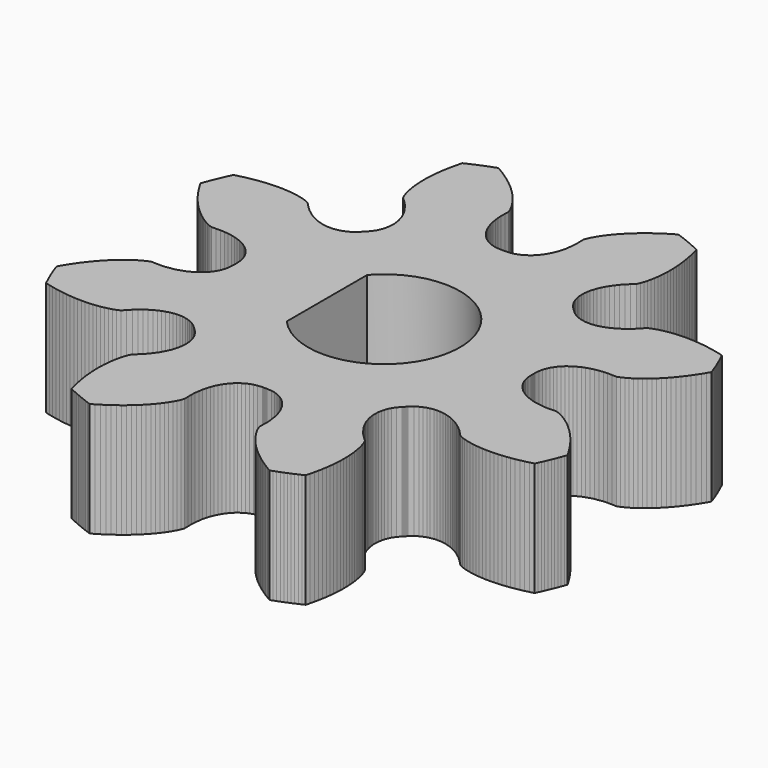
from build123d import *

# Parameters (mm, degrees)
F1_DEPTH = 3


# Not quite as in the source:
# - ends of sketch curves that miss each other by under 0.0002 mm in the source are joined


with BuildPart() as f1:
    # F0 (on Top) → F1 (new body)
    with BuildSketch(Plane.XY):
        Polygon((3.91873, -0.01261), (3.91875, 0), (3.91873, 0.01261), (3.918669, 0.02522), (3.918567, 0.037829), (3.918425, 0.050438), (3.918243, 0.063047), (3.927022, 0.180894), (3.946465, 0.280905), (3.974611, 0.359921), (4.009085, 0.438851), (4.050739, 0.504778), (4.097447, 0.573512), (4.150796, 0.631412), (4.209027, 0.689888), (4.273539, 0.739418), (4.342741, 0.789047), (4.418306, 0.828977), (4.498112, 0.870334), (4.584187, 0.902056), (4.674962, 0.93187), (4.771145, 0.955731), (4.873257, 0.970539), (4.979177, 0.986368), (5.091067, 0.991698), (5.208217, 0.989239), (5.32907, 0.986364), (5.410163, 1.016651), (5.489651, 1.055105), (5.56805, 1.098614), (5.64541, 1.146577), (5.721741, 1.198614), (5.797032, 1.254457), (5.87126, 1.313903), (5.944393, 1.376794), (6.016393, 1.443001), (6.08722, 1.512416), (6.15683, 1.584946), (6.225176, 1.660508), (6.292211, 1.739031), (6.357886, 1.820446), (6.42215, 1.904693), (6.484952, 1.991715), (6.546241, 2.081459), (6.605965, 2.173872), (6.664072, 2.268905), (6.72051, 2.36651), (6.694499, 2.43912), (6.667703, 2.511445), (6.640127, 2.583475), (6.611771, 2.655203), (6.582642, 2.726619), (6.5527401565, 2.797716063), (6.5220715212, 2.8684861381), (6.4906377963, 2.9389182162), (6.4584439317, 3.0090073474), (6.4254934628, 3.0787429253), (6.3165686129, 3.1078523901), (6.2082822804, 3.1339630151), (6.100705176, 3.1570776287), (5.9939087176, 3.1771983522), (5.8879671512, 3.1943244784), (5.782954016, 3.2084545932), (5.6789456796, 3.219584454), (5.5760206307, 3.2277076967), (5.474262308, 3.2328101792), (5.3737541501, 3.234874931), (5.2745880809, 3.2338764962), (5.176860974, 3.2297802266), (5.0806774812, 3.222538039), (4.9861556894, 3.2120855865), (4.8934299487, 3.1983337739), (4.8026600654, 3.1811553217), (4.7140433223, 3.1603685037), (4.6278413488, 3.1356975481), (4.5444437608, 3.1066821284), (4.4656862075, 3.0707568613), (4.3822631637, 2.9832679535), (4.3011643799, 2.8986916185), (4.218277323, 2.8233423199), (4.1321877795, 2.7596383629), (4.0495128546, 2.6979051124), (3.9646289282, 2.6467657358), (3.8793596285, 2.6036597993), (3.796064571, 2.5652264244), (3.7103893921, 2.5380388758), (3.6287220944, 2.5128411257), (3.5446958885, 2.4990009246), (3.464056017, 2.4884070508), (3.3815317058, 2.488580292), (3.3028667835, 2.491798335), (3.2212369625, 2.5073730689), (3.1451657079, 2.5245366718), (3.0649769705, 2.5559718109), (2.9892019936, 2.5919423328), (2.9047352601, 2.648912512), (2.8151971569, 2.7260352344), (2.8064099409, 2.7350798372), (2.7975944407, 2.7440961558), (2.7887506561, 2.7530841901), (2.7798771732, 2.7620439401), (2.7709746988, 2.7709746988), (2.7620439401, 2.7798771732), (2.7530841901, 2.7887506561), (2.7440961558, 2.7975944407), (2.7350798372, 2.8064099409), (2.7260352344, 2.8151971569), (2.648912512, 2.9047352601), (2.5919423328, 2.9892019936), (2.5559718109, 3.0649769705), (2.5245366718, 3.1451657079), (2.5073730689, 3.2212369625), (2.491798335, 3.3028667835), (2.488580292, 3.3815317058), (2.4884070508, 3.464056017), (2.4990009246, 3.5446958885), (2.5128411257, 3.6287220944), (2.5380388758, 3.7103893921), (2.5652264244, 3.796064571), (2.6036597993, 3.8793596285), (2.6467657358, 3.9646289282), (2.6979051124, 4.0495128546), (2.7596383629, 4.1321877795), (2.8233423199, 4.218277323), (2.8986916185, 4.3011643799), (2.9832679535, 4.3822631637), (3.0707568613, 4.4656862075), (3.1066821284, 4.5444437608), (3.1356975481, 4.6278413488), (3.1603685037, 4.7140433223), (3.1811553217, 4.8026600654), (3.1983337739, 4.8934299487), (3.2120855865, 4.9861556894), (3.222538039, 5.0806774812), (3.2297802266, 5.176860974), (3.2338764962, 5.2745880809), (3.234874931, 5.3737541501), (3.2328101792, 5.474262308), (3.2277076967, 5.5760206307), (3.219584454, 5.6789456796), (3.2084545932, 5.782954016), (3.1943244784, 5.8879671512), (3.1771983522, 5.9939087176), (3.1570776287, 6.100705176), (3.1339630151, 6.2082822804), (3.1078523901, 6.3165686129), (3.0787429253, 6.4254934628), (3.0090073474, 6.4584439317), (2.9389182162, 6.4906377963), (2.8684861381, 6.5220715212), (2.797716063, 6.5527401565), (2.7266200117, 6.5826415809), (2.655203, 6.611771), (2.583475, 6.640127), (2.511445, 6.667703), (2.43912, 6.694499), (2.36651, 6.72051), (2.268905, 6.664072), (2.173872, 6.605965), (2.081459, 6.546241), (1.991715, 6.484952), (1.904693, 6.42215), (1.820446, 6.357886), (1.739031, 6.292211), (1.660508, 6.225176), (1.584946, 6.15683), (1.512416, 6.08722), (1.443001, 6.016393), (1.376794, 5.944393), (1.313903, 5.87126), (1.254457, 5.797032), (1.198614, 5.721741), (1.146577, 5.64541), (1.098614, 5.56805), (1.055105, 5.489651), (1.016651, 5.410163), (0.986364, 5.32907), (0.989239, 5.208217), (0.991698, 5.091067), (0.986368, 4.979177), (0.970539, 4.873257), (0.955731, 4.771145), (0.93187, 4.674962), (0.902056, 4.584187), (0.870334, 4.498112), (0.828977, 4.418306), (0.789047, 4.342741), (0.739418, 4.273539), (0.689888, 4.209027), (0.631412, 4.150796), (0.573512, 4.097447), (0.504778, 4.050739), (0.438851, 4.009085), (0.359921, 3.974611), (0.280905, 3.946465), (0.180894, 3.927022), (0.063047, 3.918243), (0.050438, 3.918425), (0.037829, 3.918567), (0.02522, 3.918669), (0.01261, 3.91873), (0, 3.91875), (-0.01261, 3.91873), (-0.02522, 3.918669), (-0.037829, 3.918567), (-0.050438, 3.918425), (-0.063047, 3.918243), (-0.180894, 3.927022), (-0.280905, 3.946465), (-0.359921, 3.974611), (-0.438851, 4.009085), (-0.504778, 4.050739), (-0.573512, 4.097447), (-0.631412, 4.150796), (-0.689888, 4.209027), (-0.739418, 4.273539), (-0.789047, 4.342741), (-0.828977, 4.418306), (-0.870334, 4.498112), (-0.902056, 4.584187), (-0.93187, 4.674962), (-0.955731, 4.771145), (-0.970539, 4.873257), (-0.986368, 4.979177), (-0.991698, 5.091067), (-0.989239, 5.208217), (-0.986364, 5.32907), (-1.016651, 5.410163), (-1.055105, 5.489651), (-1.098614, 5.56805), (-1.146577, 5.64541), (-1.198614, 5.721741), (-1.254457, 5.797032), (-1.313903, 5.87126), (-1.376794, 5.944393), (-1.443001, 6.016393), (-1.512416, 6.08722), (-1.584946, 6.15683), (-1.660508, 6.225176), (-1.739031, 6.292211), (-1.820446, 6.357886), (-1.904693, 6.42215), (-1.991715, 6.484952), (-2.081459, 6.546241), (-2.173872, 6.605965), (-2.268905, 6.664072), (-2.36651, 6.72051), (-2.43912, 6.694499), (-2.511445, 6.667703), (-2.583475, 6.640127), (-2.655203, 6.611771), (-2.726619, 6.582642), (-2.797716063, 6.5527401565), (-2.8684861381, 6.5220715212), (-2.9389182162, 6.4906377963), (-3.0090073474, 6.4584439317), (-3.0787429253, 6.4254934628), (-3.1078523901, 6.3165686129), (-3.1339630151, 6.2082822804), (-3.1570776287, 6.100705176), (-3.1771983522, 5.9939087176), (-3.1943244784, 5.8879671512), (-3.2084545932, 5.782954016), (-3.219584454, 5.6789456796), (-3.2277076967, 5.5760206307), (-3.2328101792, 5.474262308), (-3.234874931, 5.3737541501), (-3.2338764962, 5.2745880809), (-3.2297802266, 5.176860974), (-3.222538039, 5.0806774812), (-3.2120855865, 4.9861556894), (-3.1983337739, 4.8934299487), (-3.1811553217, 4.8026600654), (-3.1603685037, 4.7140433223), (-3.1356975481, 4.6278413488), (-3.1066821284, 4.5444437608), (-3.0707568613, 4.4656862075), (-2.9832679535, 4.3822631637), (-2.8986916185, 4.3011643799), (-2.8233423199, 4.218277323), (-2.7596383629, 4.1321877795), (-2.6979051124, 4.0495128546), (-2.6467657358, 3.9646289282), (-2.6036597993, 3.8793596285), (-2.5652264244, 3.796064571), (-2.5380388758, 3.7103893921), (-2.5128411257, 3.6287220944), (-2.4990009246, 3.5446958885), (-2.4884070508, 3.464056017), (-2.488580292, 3.3815317058), (-2.491798335, 3.3028667835), (-2.5073730689, 3.2212369625), (-2.5245366718, 3.1451657079), (-2.5559718109, 3.0649769705), (-2.5919423328, 2.9892019936), (-2.648912512, 2.9047352601), (-2.7260352344, 2.8151971569), (-2.7350798372, 2.8064099409), (-2.7440961558, 2.7975944407), (-2.7530841901, 2.7887506561), (-2.7620439401, 2.7798771732), (-2.7709746988, 2.7709746988), (-2.7798771732, 2.7620439401), (-2.7887506561, 2.7530841901), (-2.7975944407, 2.7440961558), (-2.8064099409, 2.7350798372), (-2.8151971569, 2.7260352344), (-2.9047352601, 2.648912512), (-2.9892019936, 2.5919423328), (-3.0649769705, 2.5559718109), (-3.1451657079, 2.5245366718), (-3.2212369625, 2.5073730689), (-3.3028667835, 2.491798335), (-3.3815317058, 2.488580292), (-3.464056017, 2.4884070508), (-3.5446958885, 2.4990009246), (-3.6287220944, 2.5128411257), (-3.7103893921, 2.5380388758), (-3.796064571, 2.5652264244), (-3.8793596285, 2.6036597993), (-3.9646289282, 2.6467657358), (-4.0495128546, 2.6979051124), (-4.1321877795, 2.7596383629), (-4.218277323, 2.8233423199), (-4.3011643799, 2.8986916185), (-4.3822631637, 2.9832679535), (-4.4656862075, 3.0707568613), (-4.5444437608, 3.1066821284), (-4.6278413488, 3.1356975481), (-4.7140433223, 3.1603685037), (-4.8026600654, 3.1811553217), (-4.8934299487, 3.1983337739), (-4.9861556894, 3.2120855865), (-5.0806774812, 3.222538039), (-5.176860974, 3.2297802266), (-5.2745880809, 3.2338764962), (-5.3737541501, 3.234874931), (-5.474262308, 3.2328101792), (-5.5760206307, 3.2277076967), (-5.6789456796, 3.219584454), (-5.782954016, 3.2084545932), (-5.8879671512, 3.1943244784), (-5.9939087176, 3.1771983522), (-6.100705176, 3.1570776287), (-6.2082822804, 3.1339630151), (-6.3165686129, 3.1078523901), (-6.4254934628, 3.0787429253), (-6.4584439317, 3.0090073474), (-6.4906377963, 2.9389182162), (-6.5220715212, 2.8684861381), (-6.5527401565, 2.797716063), (-6.5826415809, 2.7266200117), (-6.611771, 2.655203), (-6.640127, 2.583475), (-6.667703, 2.511445), (-6.694499, 2.43912), (-6.72051, 2.36651), (-6.664072, 2.268905), (-6.605965, 2.173872), (-6.546241, 2.081459), (-6.484952, 1.991715), (-6.42215, 1.904693), (-6.357886, 1.820446), (-6.292211, 1.739031), (-6.225176, 1.660508), (-6.15683, 1.584946), (-6.08722, 1.512416), (-6.016393, 1.443001), (-5.944393, 1.376794), (-5.87126, 1.313903), (-5.797032, 1.254457), (-5.721741, 1.198614), (-5.64541, 1.146577), (-5.56805, 1.098614), (-5.489651, 1.055105), (-5.410163, 1.016651), (-5.32907, 0.986364), (-5.208217, 0.989239), (-5.091067, 0.991698), (-4.979177, 0.986368), (-4.873257, 0.970539), (-4.771145, 0.955731), (-4.674962, 0.93187), (-4.584187, 0.902056), (-4.498112, 0.870334), (-4.418306, 0.828977), (-4.342741, 0.789047), (-4.273539, 0.739418), (-4.209027, 0.689888), (-4.150796, 0.631412), (-4.097447, 0.573512), (-4.050739, 0.504778), (-4.009085, 0.438851), (-3.974611, 0.359921), (-3.946465, 0.280905), (-3.927022, 0.180894), (-3.918243, 0.063047), (-3.918425, 0.050438), (-3.918567, 0.037829), (-3.918669, 0.02522), (-3.91873, 0.01261), (-3.91875, 0), (-3.91873, -0.01261), (-3.918669, -0.02522), (-3.918567, -0.037829), (-3.918425, -0.050438), (-3.918243, -0.063047), (-3.927022, -0.180894), (-3.946465, -0.280905), (-3.974611, -0.359921), (-4.009085, -0.438851), (-4.050739, -0.504778), (-4.097447, -0.573512), (-4.150796, -0.631412), (-4.209027, -0.689888), (-4.273539, -0.739418), (-4.342741, -0.789047), (-4.418306, -0.828977), (-4.498112, -0.870334), (-4.584187, -0.902056), (-4.674962, -0.93187), (-4.771145, -0.955731), (-4.873257, -0.970539), (-4.979177, -0.986368), (-5.091067, -0.991698), (-5.208217, -0.989239), (-5.32907, -0.986364), (-5.410163, -1.016651), (-5.489651, -1.055105), (-5.56805, -1.098614), (-5.64541, -1.146577), (-5.721741, -1.198614), (-5.797032, -1.254457), (-5.87126, -1.313903), (-5.944393, -1.376794), (-6.016393, -1.443001), (-6.08722, -1.512416), (-6.15683, -1.584946), (-6.225176, -1.660508), (-6.292211, -1.739031), (-6.357886, -1.820446), (-6.42215, -1.904693), (-6.484952, -1.991715), (-6.546241, -2.081459), (-6.605965, -2.173872), (-6.664072, -2.268905), (-6.72051, -2.36651), (-6.694499, -2.43912), (-6.667703, -2.511445), (-6.640127, -2.583475), (-6.611771, -2.655203), (-6.582642, -2.726619), (-6.5527401565, -2.797716063), (-6.5220715212, -2.8684861381), (-6.4906377963, -2.9389182162), (-6.4584439317, -3.0090073474), (-6.4254934628, -3.0787429253), (-6.3165686129, -3.1078523901), (-6.2082822804, -3.1339630151), (-6.100705176, -3.1570776287), (-5.9939087176, -3.1771983522), (-5.8879671512, -3.1943244784), (-5.782954016, -3.2084545932), (-5.6789456796, -3.219584454), (-5.5760206307, -3.2277076967), (-5.474262308, -3.2328101792), (-5.3737541501, -3.234874931), (-5.2745880809, -3.2338764962), (-5.176860974, -3.2297802266), (-5.0806774812, -3.222538039), (-4.9861556894, -3.2120855865), (-4.8934299487, -3.1983337739), (-4.8026600654, -3.1811553217), (-4.7140433223, -3.1603685037), (-4.6278413488, -3.1356975481), (-4.5444437608, -3.1066821284), (-4.4656862075, -3.0707568613), (-4.3822631637, -2.9832679535), (-4.3011643799, -2.8986916185), (-4.218277323, -2.8233423199), (-4.1321877795, -2.7596383629), (-4.0495128546, -2.6979051124), (-3.9646289282, -2.6467657358), (-3.8793596285, -2.6036597993), (-3.796064571, -2.5652264244), (-3.7103893921, -2.5380388758), (-3.6287220944, -2.5128411257), (-3.5446958885, -2.4990009246), (-3.464056017, -2.4884070508), (-3.3815317058, -2.488580292), (-3.3028667835, -2.491798335), (-3.2212369625, -2.5073730689), (-3.1451657079, -2.5245366718), (-3.0649769705, -2.5559718109), (-2.9892019936, -2.5919423328), (-2.9047352601, -2.648912512), (-2.8151971569, -2.7260352344), (-2.8064099409, -2.7350798372), (-2.7975944407, -2.7440961558), (-2.7887506561, -2.7530841901), (-2.7798771732, -2.7620439401), (-2.7709746988, -2.7709746988), (-2.7620439401, -2.7798771732), (-2.7530841901, -2.7887506561), (-2.7440961558, -2.7975944407), (-2.7350798372, -2.8064099409), (-2.7260352344, -2.8151971569), (-2.648912512, -2.9047352601), (-2.5919423328, -2.9892019936), (-2.5559718109, -3.0649769705), (-2.5245366718, -3.1451657079), (-2.5073730689, -3.2212369625), (-2.491798335, -3.3028667835), (-2.488580292, -3.3815317058), (-2.4884070508, -3.464056017), (-2.4990009246, -3.5446958885), (-2.5128411257, -3.6287220944), (-2.5380388758, -3.7103893921), (-2.5652264244, -3.796064571), (-2.6036597993, -3.8793596285), (-2.6467657358, -3.9646289282), (-2.6979051124, -4.0495128546), (-2.7596383629, -4.1321877795), (-2.8233423199, -4.218277323), (-2.8986916185, -4.3011643799), (-2.9832679535, -4.3822631637), (-3.0707568613, -4.4656862075), (-3.1066821284, -4.5444437608), (-3.1356975481, -4.6278413488), (-3.1603685037, -4.7140433223), (-3.1811553217, -4.8026600654), (-3.1983337739, -4.8934299487), (-3.2120855865, -4.9861556894), (-3.222538039, -5.0806774812), (-3.2297802266, -5.176860974), (-3.2338764962, -5.2745880809), (-3.234874931, -5.3737541501), (-3.2328101792, -5.474262308), (-3.2277076967, -5.5760206307), (-3.219584454, -5.6789456796), (-3.2084545932, -5.782954016), (-3.1943244784, -5.8879671512), (-3.1771983522, -5.9939087176), (-3.1570776287, -6.100705176), (-3.1339630151, -6.2082822804), (-3.1078523901, -6.3165686129), (-3.0787429253, -6.4254934628), (-3.0090073474, -6.4584439317), (-2.9389182162, -6.4906377963), (-2.8684861381, -6.5220715212), (-2.797716063, -6.5527401565), (-2.7266200117, -6.5826415809), (-2.655203, -6.611771), (-2.583475, -6.640127), (-2.511445, -6.667703), (-2.43912, -6.694499), (-2.36651, -6.72051), (-2.268905, -6.664072), (-2.173872, -6.605965), (-2.081459, -6.546241), (-1.991715, -6.484952), (-1.904693, -6.42215), (-1.820446, -6.357886), (-1.739031, -6.292211), (-1.660508, -6.225176), (-1.584946, -6.15683), (-1.512416, -6.08722), (-1.443001, -6.016393), (-1.376794, -5.944393), (-1.313903, -5.87126), (-1.254457, -5.797032), (-1.198614, -5.721741), (-1.146577, -5.64541), (-1.098614, -5.56805), (-1.055105, -5.489651), (-1.016651, -5.410163), (-0.986364, -5.32907), (-0.989239, -5.208217), (-0.991698, -5.091067), (-0.986368, -4.979177), (-0.970539, -4.873257), (-0.955731, -4.771145), (-0.93187, -4.674962), (-0.902056, -4.584187), (-0.870334, -4.498112), (-0.828977, -4.418306), (-0.789047, -4.342741), (-0.739418, -4.273539), (-0.689888, -4.209027), (-0.631412, -4.150796), (-0.573512, -4.097447), (-0.504778, -4.050739), (-0.438851, -4.009085), (-0.359921, -3.974611), (-0.280905, -3.946465), (-0.180894, -3.927022), (-0.063047, -3.918243), (-0.050438, -3.918425), (-0.037829, -3.918567), (-0.02522, -3.918669), (-0.01261, -3.91873), (0, -3.91875), (0.01261, -3.91873), (0.02522, -3.918669), (0.037829, -3.918567), (0.050438, -3.918425), (0.063047, -3.918243), (0.180894, -3.927022), (0.280905, -3.946465), (0.359921, -3.974611), (0.438851, -4.009085), (0.504778, -4.050739), (0.573512, -4.097447), (0.631412, -4.150796), (0.689888, -4.209027), (0.739418, -4.273539), (0.789047, -4.342741), (0.828977, -4.418306), (0.870334, -4.498112), (0.902056, -4.584187), (0.93187, -4.674962), (0.955731, -4.771145), (0.970539, -4.873257), (0.986368, -4.979177), (0.991698, -5.091067), (0.989239, -5.208217), (0.986364, -5.32907), (1.016651, -5.410163), (1.055105, -5.489651), (1.098614, -5.56805), (1.146577, -5.64541), (1.198614, -5.721741), (1.254457, -5.797032), (1.313903, -5.87126), (1.376794, -5.944393), (1.443001, -6.016393), (1.512416, -6.08722), (1.584946, -6.15683), (1.660508, -6.225176), (1.739031, -6.292211), (1.820446, -6.357886), (1.904693, -6.42215), (1.991715, -6.484952), (2.081459, -6.546241), (2.173872, -6.605965), (2.268905, -6.664072), (2.36651, -6.72051), (2.43912, -6.694499), (2.511445, -6.667703), (2.583475, -6.640127), (2.655203, -6.611771), (2.726619, -6.582642), (2.797716063, -6.5527401565), (2.8684861381, -6.5220715212), (2.9389182162, -6.4906377963), (3.0090073474, -6.4584439317), (3.0787429253, -6.4254934628), (3.1078523901, -6.3165686129), (3.1339630151, -6.2082822804), (3.1570776287, -6.100705176), (3.1771983522, -5.9939087176), (3.1943244784, -5.8879671512), (3.2084545932, -5.782954016), (3.219584454, -5.6789456796), (3.2277076967, -5.5760206307), (3.2328101792, -5.474262308), (3.234874931, -5.3737541501), (3.2338764962, -5.2745880809), (3.2297802266, -5.176860974), (3.222538039, -5.0806774812), (3.2120855865, -4.9861556894), (3.1983337739, -4.8934299487), (3.1811553217, -4.8026600654), (3.1603685037, -4.7140433223), (3.1356975481, -4.6278413488), (3.1066821284, -4.5444437608), (3.0707568613, -4.4656862075), (2.9832679535, -4.3822631637), (2.8986916185, -4.3011643799), (2.8233423199, -4.218277323), (2.7596383629, -4.1321877795), (2.6979051124, -4.0495128546), (2.6467657358, -3.9646289282), (2.6036597993, -3.8793596285), (2.5652264244, -3.796064571), (2.5380388758, -3.7103893921), (2.5128411257, -3.6287220944), (2.4990009246, -3.5446958885), (2.4884070508, -3.464056017), (2.488580292, -3.3815317058), (2.491798335, -3.3028667835), (2.5073730689, -3.2212369625), (2.5245366718, -3.1451657079), (2.5559718109, -3.0649769705), (2.5919423328, -2.9892019936), (2.648912512, -2.9047352601), (2.7260352344, -2.8151971569), (2.7350798372, -2.8064099409), (2.7440961558, -2.7975944407), (2.7530841901, -2.7887506561), (2.7620439401, -2.7798771732), (2.7709746988, -2.7709746988), (2.7798771732, -2.7620439401), (2.7887506561, -2.7530841901), (2.7975944407, -2.7440961558), (2.8064099409, -2.7350798372), (2.8151971569, -2.7260352344), (2.9047352601, -2.648912512), (2.9892019936, -2.5919423328), (3.0649769705, -2.5559718109), (3.1451657079, -2.5245366718), (3.2212369625, -2.5073730689), (3.3028667835, -2.491798335), (3.3815317058, -2.488580292), (3.464056017, -2.4884070508), (3.5446958885, -2.4990009246), (3.6287220944, -2.5128411257), (3.7103893921, -2.5380388758), (3.796064571, -2.5652264244), (3.8793596285, -2.6036597993), (3.9646289282, -2.6467657358), (4.0495128546, -2.6979051124), (4.1321877795, -2.7596383629), (4.218277323, -2.8233423199), (4.3011643799, -2.8986916185), (4.3822631637, -2.9832679535), (4.4656862075, -3.0707568613), (4.5444437608, -3.1066821284), (4.6278413488, -3.1356975481), (4.7140433223, -3.1603685037), (4.8026600654, -3.1811553217), (4.8934299487, -3.1983337739), (4.9861556894, -3.2120855865), (5.0806774812, -3.222538039), (5.176860974, -3.2297802266), (5.2745880809, -3.2338764962), (5.3737541501, -3.234874931), (5.474262308, -3.2328101792), (5.5760206307, -3.2277076967), (5.6789456796, -3.219584454), (5.782954016, -3.2084545932), (5.8879671512, -3.1943244784), (5.9939087176, -3.1771983522), (6.100705176, -3.1570776287), (6.2082822804, -3.1339630151), (6.3165686129, -3.1078523901), (6.4254934628, -3.0787429253), (6.4584439317, -3.0090073474), (6.4906377963, -2.9389182162), (6.5220715212, -2.8684861381), (6.5527401565, -2.797716063), (6.5826415809, -2.7266200117), (6.611771, -2.655203), (6.640127, -2.583475), (6.667703, -2.511445), (6.694499, -2.43912), (6.72051, -2.36651), (6.664072, -2.268905), (6.605965, -2.173872), (6.546241, -2.081459), (6.484952, -1.991715), (6.42215, -1.904693), (6.357886, -1.820446), (6.292211, -1.739031), (6.225176, -1.660508), (6.15683, -1.584946), (6.08722, -1.512416), (6.016393, -1.443001), (5.944393, -1.376794), (5.87126, -1.313903), (5.797032, -1.254457), (5.721741, -1.198614), (5.64541, -1.146577), (5.56805, -1.098614), (5.489651, -1.055105), (5.410163, -1.016651), (5.32907, -0.986364), (5.208217, -0.989239), (5.091067, -0.991698), (4.979177, -0.986368), (4.873257, -0.970539), (4.771145, -0.955731), (4.674962, -0.93187), (4.584187, -0.902056), (4.498112, -0.870334), (4.418306, -0.828977), (4.342741, -0.789047), (4.273539, -0.739418), (4.209027, -0.689888), (4.150796, -0.631412), (4.097447, -0.573512), (4.050739, -0.504778), (4.009085, -0.438851), (3.974611, -0.359921), (3.946465, -0.280905), (3.927022, -0.180894), (3.918243, -0.063047), (3.918425, -0.050438), (3.918567, -0.037829), (3.918669, -0.02522), align=None)
        with BuildLine():
            ThreePointArc((-1.5, 1.3228756555), (2, 0), (-1.5, -1.3228756555))
            Line((-1.5, -1.3228756555), (-1.5, 1.3228756555))
        make_face(mode=Mode.SUBTRACT)
    extrude(amount=F1_DEPTH)


solid = f1.part
